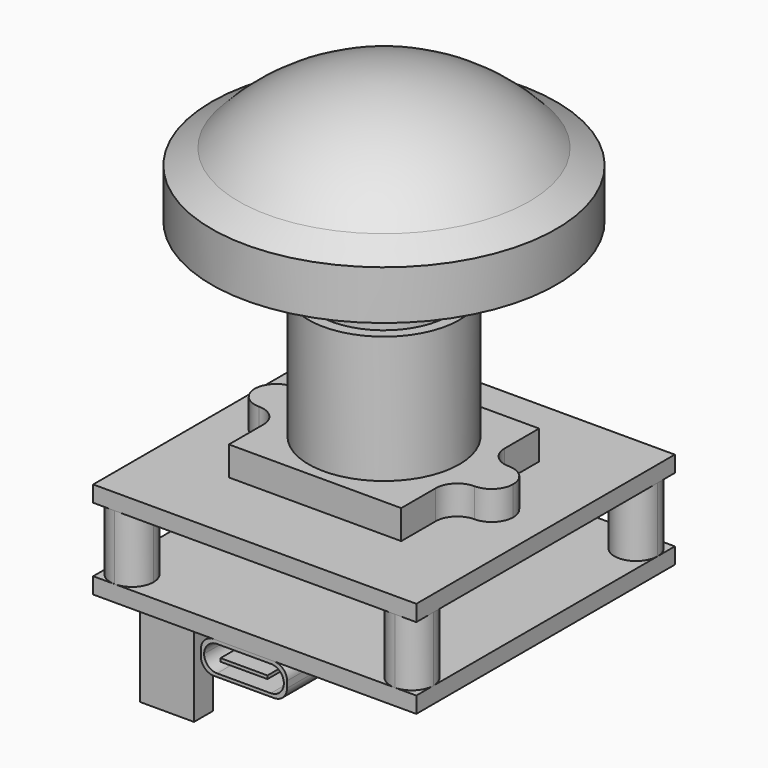
from build123d import *

# Parameters (mm, degrees)
F0_W      = 30
F0_H      = 30
F1_DEPTH  = 1.5
F2_START  = 6
F1_FACE_W = 30
F1_FACE_H = 30
F2_DEPTH  = 1.5
F3_R      = 1.25
F4_DEPTH  = 6
F5_W      = 4
F5_H      = 4
F5_R      = 7
F6_DEPTH  = 2.7
F7_R      = 1.99999
F8_DEPTH  = 14.5
F9_W      = 6
F9_H      = 5
F12_W     = 8
F12_H     = 9
F13_DEPTH = 3
F14_W     = 7.4
F14_H     = 2.4
F14_W_2   = 4.36
F14_H_2   = 0.3
F15_DEPTH = 8
F16_R     = 1.19999
F17_W     = 5
F17_H     = 2.2
F18_DEPTH = 7.5


# Not quite as in the source:
# - a fillet or chamfer is up to 0.001 mm smaller than in the source, because OpenCascade refuses the exact size


with BuildPart() as f1:
    # F0 (on Top) → F1 (new body)
    with BuildSketch(Plane.XY):
        Rectangle(F0_W, F0_H)
    extrude(amount=F1_DEPTH)


with BuildPart() as f2:
    # F1_face (on face) → F2 (new body)
    with BuildSketch(Plane.XY.offset(1.5).offset(F2_START)):
        Rectangle(F1_FACE_W, F1_FACE_H)
    extrude(amount=F2_DEPTH)


with BuildPart() as f4:
    # F3 (on face) → F4 (new body)
    with BuildSketch(Plane.XY.offset(1.5)):
        with BuildLine():
            ThreePointArc((-11, 13), (-11.5857864376, 14.4142135624), (-13, 15))
            ThreePointArc((-13, 15), (-14.4142135624, 14.4142135624), (-15, 13))
            ThreePointArc((-15, 13), (-13, 11), (-11, 13))
        make_face()
        with Locations((-13, 13)):
            Circle(F3_R, mode=Mode.SUBTRACT)
    extrude(amount=F4_DEPTH)


with BuildPart() as f4b:
    # F3 (on face) → F4, piece 2 (new body)
    with BuildSketch(Plane.XY.offset(1.5)):
        with BuildLine():
            ThreePointArc((-15, -13), (-14.4142135624, -14.4142135624), (-13, -15))
            ThreePointArc((-13, -15), (-11.5857864376, -14.4142135624), (-11, -13))
            ThreePointArc((-11, -13), (-13, -11), (-15, -13))
        make_face()
        with Locations((-13, -13)):
            Circle(F3_R, mode=Mode.SUBTRACT)
    extrude(amount=F4_DEPTH)


with BuildPart() as f4c:
    # F3 (on face) → F4, piece 3 (new body)
    with BuildSketch(Plane.XY.offset(1.5)):
        with BuildLine():
            ThreePointArc((13, -15), (14.4142135624, -14.4142135624), (15, -13))
            ThreePointArc((15, -13), (11.5857864376, -11.5857864376), (13, -15))
        make_face()
        with Locations((13, -13)):
            Circle(F3_R, mode=Mode.SUBTRACT)
    extrude(amount=F4_DEPTH)


with BuildPart() as f4d:
    # F3 (on face) → F4, piece 4 (new body)
    with BuildSketch(Plane.XY.offset(1.5)):
        with BuildLine():
            ThreePointArc((13, 15), (11.5857864376, 11.5857864376), (15, 13))
            ThreePointArc((15, 13), (14.4142135624, 14.4142135624), (13, 15))
        make_face()
        with Locations((13, 13)):
            Circle(F3_R, mode=Mode.SUBTRACT)
    extrude(amount=F4_DEPTH)


with BuildPart() as f6:
    # F5 (on face) → F6 (new body)
    with BuildSketch(Plane.XY.offset(9)):
        with Locations((-10, 0)):
            Rectangle(F5_W, F5_H)
        Polygon((-8, -8), (8, -8), (8, -2), (8, 2), (8, 8), (-8, 8), (-8, 2), (-8, -2), align=None)
        Circle(F5_R, mode=Mode.SUBTRACT)
        with Locations((10, 0)):
            Rectangle(F5_W, F5_H)
        Circle(F5_R)
    extrude(amount=F6_DEPTH)

    # F7 (radius 2 in the source; OpenCascade refuses exactly that, so slightly less here)
    f7_edges = [f6.edges().sort_by_distance(p)[0] for p in [
        (-12, 2, 10.35),
        (-12, -2, 10.35),
        (-8, 2, 10.35),
        (-8, -2, 10.35),
        (12, -2, 10.35),
        (8, -2, 10.35),
        (8, 2, 10.35),
        (12, 2, 10.35),
    ]]
    fillet(f7_edges, radius=F7_R)

    # F5 (on face) → F8 (join)
    with BuildSketch(Plane.XY.offset(9)):
        Circle(F5_R)
    extrude(amount=F8_DEPTH)


with BuildPart() as f10:
    # F9 (on Front) → F10 (revolve)
    with BuildSketch(Plane.XZ):
        with BuildLine():
            Line((-13.5, 35.3), (0, 35.3))
            Line((0, 35.3), (0, 41.3))
            ThreePointArc((0, 41.3), (-7.3866433513, 39.7324475405), (-13.5, 35.3))
        make_face()
    revolve(axis=Axis((0, 0, 25.3), (0, 0, -1)))


with BuildPart() as f11:
    # F9 (on Front) → F11 (revolve)
    with BuildSketch(Plane.XZ):
        Polygon((-9.3, 29.3), (0, 29.3), (0, 35.3), (-13.5, 35.3), (-16, 33.856624327), (-16, 29.3), align=None)
        Polygon((-6, 27.8), (0, 27.8), (0, 29.3), (-9.3, 29.3), (-9.3, 27.8), align=None)
        with Locations((-3, 25.3)):
            Rectangle(F9_W, F9_H)
    revolve(axis=Axis((0, 0, 25.3), (0, 0, -1)))


with BuildPart() as f13:
    # F12 (on face) → F13 (new body)
    with BuildSketch(Plane(origin=(0, 0, 0), x_dir=(1, 0, 0), z_dir=(0, 0, -1))):
        with Locations((-1, 10.5)):
            Rectangle(F12_W, F12_H)
    extrude(amount=F13_DEPTH)

    # F14 (on face) → F15 (cut)
    with BuildSketch(Plane.XZ.offset(15)):
        with Locations((-1, -1.5)):
            Rectangle(F14_W, F14_H)
        with Locations((-1, -1.5)):
            Rectangle(F14_W_2, F14_H_2, mode=Mode.SUBTRACT)
    extrude(amount=-F15_DEPTH, mode=Mode.SUBTRACT)

    # F16 (radius 1.2 in the source; OpenCascade refuses exactly that, so slightly less here)
    f16_edges = [f13.edges().sort_by_distance(p)[0] for p in [
        (-5, -10.5, -3),
        (-5, -10.5, 0),
        (3, -10.5, 0),
        (3, -10.5, -3),
        (-4.7, -11, -0.3),
        (2.7, -11, -0.3),
        (2.7, -11, -2.7),
        (-4.7, -11, -2.7),
    ]]
    fillet(f16_edges, radius=F16_R)


with BuildPart() as f18:
    # F17 (on face) → F18 (new body)
    with BuildSketch(Plane(origin=(0, 0, 0), x_dir=(1, 0, 0), z_dir=(0, 0, -1))):
        with Locations((-8.3, 13.7)):
            Rectangle(F17_W, F17_H)
    extrude(amount=F18_DEPTH)


solid = Compound([f1.part, f2.part, f4.part, f4b.part, f4c.part, f4d.part, f6.part, f10.part, f11.part, f13.part, f18.part])
